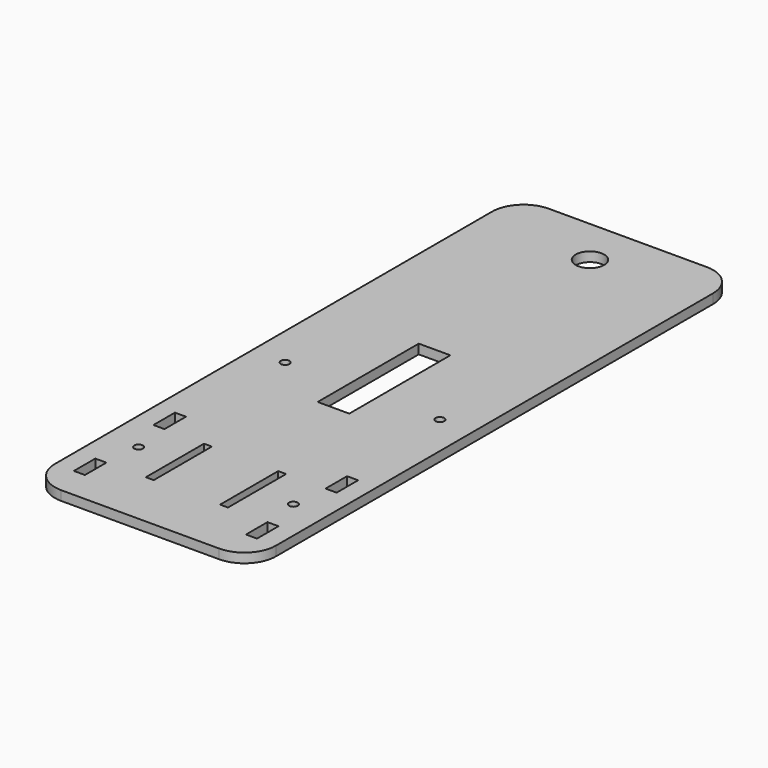
from build123d import *

# Parameters (mm, degrees)
F0_R     = 1.375
F0_R_2   = 4.5
F0_W     = 40
F0_H     = 10
F0_W_2   = 10
F0_H_2   = 35
F0_W_3   = 15
F0_H_3   = 2
F0_W_4   = 2
F0_W_5   = 5.5
F0_H_4   = 11.5
F0_R_3   = 1
F1_DEPTH = 3


# Not quite as in the source:
# - a feature names something its author has since deleted; it is built from what else it names


with BuildPart() as f1:
    # F0 (on Top) → F1 (new body)
    with BuildSketch(Plane.XY):
        with BuildLine():
            Line((25, 96.5), (-25, 96.5))
            ThreePointArc((-25, 96.5), (-32.0710678119, 93.5710678119), (-35, 86.5))
            Line((-35, 86.5), (-35, -86.5))
            ThreePointArc((-35, -86.5), (-32.0710678119, -93.5710678119), (-25, -96.5))
            Line((-25, -96.5), (25, -96.5))
            ThreePointArc((25, -96.5), (32.0710678119, -93.5710678119), (35, -86.5))
            Line((35, -86.5), (35, 86.5))
            ThreePointArc((35, 86.5), (32.0710678119, 93.5710678119), (25, 96.5))
        make_face()
        Polygon((-29, -86.5), (-29, -78), (-29, -55), (-29, -46.5), (-25.5, -46.5), (-25.5, -55), (-18.5, -55), (-13, -55), (-10.5, -55), (-10.5, -66.5), (-10.5, -78), (-10.5, -86.5), (-25.5, -86.5), align=None, mode=Mode.SUBTRACT)
        with Locations((-24.5, -8.5)):
            Circle(F0_R, mode=Mode.SUBTRACT)
        Polygon((10.5, -78), (10.5, -66.5), (10.5, -55), (13, -55), (18.5, -55), (24.5, -55), (25.5, -55), (25.5, -46.5), (29, -46.5), (29, -55), (29, -78), (29, -86.5), (25.5, -86.5), (10.5, -86.5), align=None, mode=Mode.SUBTRACT)
        with BuildLine():
            ThreePointArc((25.875, -8.5), (25.4722718241, -9.4722718241), (24.5, -9.875))
            ThreePointArc((24.5, -9.875), (23.5277281759, -7.5277281759), (25.875, -8.5))
        make_face(mode=Mode.SUBTRACT)
        with BuildLine():
            ThreePointArc((26, -30), (25.5980762114, -31.5), (24.5, -32.5980762114))
            ThreePointArc((24.5, -32.5980762114), (23.1822131445, -32.9944612821), (21.8260869565, -32.7607839768))
            ThreePointArc((21.8260869565, -32.7607839768), (0, -52), (-21.8260869565, -32.7607839768))
            ThreePointArc((-21.8260869565, -32.7607839768), (-26, -30), (-21.8260869565, -27.2392160232))
            ThreePointArc((-21.8260869565, -27.2392160232), (-16.3398685927, -15.268785034), (-5, -8.5757147144))
            Line((-5, -8.5757147144), (-5, -5.5))
            Line((-5, -5.5), (-14, -5.5))
            Line((-14, -5.5), (-14, -8.5))
            ThreePointArc((-14, -8.5), (-17, -11.5), (-20, -8.5))
            Line((-20, -8.5), (-20, -5.5))
            Line((-20, -5.5), (-30, -5.5))
            Line((-30, -5.5), (-32, -5.5))
            Line((-32, -5.5), (-32, 6.5))
            Line((-32, 6.5), (-32, 41.5))
            Line((-32, 41.5), (-32, 53.5))
            Line((-32, 53.5), (-30, 53.5))
            Line((-30, 53.5), (-30, 56.5))
            ThreePointArc((-30, 56.5), (-27, 59.5), (-24, 56.5))
            Line((-24, 56.5), (-24, 53.5))
            Line((-24, 53.5), (-20, 53.5))
            Line((-20, 53.5), (20, 53.5))
            Line((20, 53.5), (32, 53.5))
            Line((32, 53.5), (32, 41.5))
            Line((32, 41.5), (32, 6.5))
            Line((32, 6.5), (32, -5.5))
            Line((32, -5.5), (20, -5.5))
            Line((20, -5.5), (5, -5.5))
            Line((5, -5.5), (5, -8.5757147144))
            ThreePointArc((5, -8.5757147144), (16.3398685927, -15.268785034), (21.8260869565, -27.2392160232))
            ThreePointArc((21.8260869565, -27.2392160232), (23.1822131445, -27.0055387179), (24.5, -27.4019237886))
            ThreePointArc((24.5, -27.4019237886), (25.5980762114, -28.5), (26, -30))
        make_face(mode=Mode.SUBTRACT)
        with Locations((0, 81.5)):
            Circle(F0_R_2, mode=Mode.SUBTRACT)
        Polygon((5, 20), (5, 6.5), (20, 6.5), (20, 41.5), (-20, 41.5), (-20, 6.5), (-5, 6.5), (-5, 20), align=None)
        with BuildLine():
            ThreePointArc((-20, -30), (0, -50), (20, -30))
            ThreePointArc((20, -30), (15.8113883008, -17.7525512861), (5, -10.635083269))
            Line((5, -10.635083269), (5, -20))
            Line((5, -20), (-5, -20))
            Line((-5, -20), (-5, -10.635083269))
            ThreePointArc((-5, -10.635083269), (-15.8113883008, -17.7525512861), (-20, -30))
        make_face()
        with Locations((0, 46.5)):
            Rectangle(F0_W, F0_H)
        with Locations((-25, 24)):
            Rectangle(F0_W_2, F0_H_2)
        with Locations((25, 24)):
            Rectangle(F0_W_2, F0_H_2)
        Polygon((-29, -55), (-29, -78), (-25.5, -78), (-18.5, -78), (-18.5, -66.5), (-18.5, -55), (-25.5, -55), align=None)
        with Locations((-24.5, -66.5)):
            Circle(F0_R, mode=Mode.SUBTRACT)
        with BuildLine():
            Line((23.125, -66.5), (18.5, -66.5))
            Line((18.5, -66.5), (18.5, -78))
            Line((18.5, -78), (25.5, -78))
            Line((25.5, -78), (29, -78))
            Line((29, -78), (29, -55))
            Line((29, -55), (25.5, -55))
            Line((25.5, -55), (24.5, -55))
            Line((24.5, -55), (24.5, -65.125))
            ThreePointArc((24.5, -65.125), (25.4722718241, -65.5277281759), (25.875, -66.5))
            ThreePointArc((25.875, -66.5), (24.5, -67.875), (23.125, -66.5))
        make_face()
        with Locations((-12.5, 1.5)):
            Rectangle(F0_W_3, F0_H)
        with Locations((12.5, 1.5)):
            Rectangle(F0_W_3, F0_H)
        Polygon((-18.5, -78), (-25.5, -78), (-25.5, -86.5), (-10.5, -86.5), (-10.5, -78), (-13, -78), align=None)
        Polygon((13, -78), (10.5, -78), (10.5, -86.5), (25.5, -86.5), (25.5, -78), (18.5, -78), align=None)
        with BuildLine():
            ThreePointArc((-21.8260869565, -32.7607839768), (0, -52), (21.8260869565, -32.7607839768))
            ThreePointArc((21.8260869565, -32.7607839768), (20.4978270313, -31.6550318531), (20, -30))
            ThreePointArc((20, -30), (0, -50), (-20, -30))
            ThreePointArc((-20, -30), (-20.4978270313, -31.6550318531), (-21.8260869565, -32.7607839768))
        make_face()
        with Locations((25, 46.5)):
            Rectangle(F0_W_2, F0_H)
        with Locations((-25, 46.5)):
            Rectangle(F0_W_2, F0_H)
        with Locations((-25, 1.5)):
            Rectangle(F0_W_2, F0_H)
        with Locations((25, 1.5)):
            Rectangle(F0_W_2, F0_H)
        with Locations((0, 52.5)):
            Rectangle(F0_W, F0_H_3)
        with Locations((31, 24)):
            Rectangle(F0_W_4, F0_H_2)
        with Locations((-31, 24)):
            Rectangle(F0_W_4, F0_H_2)
        with BuildLine():
            Line((18.5, -55), (18.5, -66.5))
            Line((18.5, -66.5), (23.125, -66.5))
            ThreePointArc((23.125, -66.5), (23.5277281759, -65.5277281759), (24.5, -65.125))
            Line((24.5, -65.125), (24.5, -55))
            Line((24.5, -55), (18.5, -55))
        make_face()
        with Locations((-15.75, -72.25)):
            Rectangle(F0_W_5, F0_H_4)
        with Locations((-15.75, -60.75)):
            Rectangle(F0_W_5, F0_H_4)
        with Locations((15.75, -72.25)):
            Rectangle(F0_W_5, F0_H_4)
        with Locations((15.75, -60.75)):
            Rectangle(F0_W_5, F0_H_4)
        with BuildLine():
            ThreePointArc((-5, -8.5757147144), (-16.3398685927, -15.268785034), (-21.8260869565, -27.2392160232))
            ThreePointArc((-21.8260869565, -27.2392160232), (-20.4978270313, -28.3449681469), (-20, -30))
            ThreePointArc((-20, -30), (-15.8113883008, -17.7525512861), (-5, -10.635083269))
            Line((-5, -10.635083269), (-5, -8.5757147144))
        make_face()
        with BuildLine():
            ThreePointArc((20, -30), (20.4978270313, -28.3449681469), (21.8260869565, -27.2392160232))
            ThreePointArc((21.8260869565, -27.2392160232), (16.3398685927, -15.268785034), (5, -8.5757147144))
            Line((5, -8.5757147144), (5, -10.635083269))
            ThreePointArc((5, -10.635083269), (15.8113883008, -17.7525512861), (20, -30))
        make_face()
        Polygon((30, 41.5), (32, 41.5), (32, 53.5), (20, 53.5), (20, 51.5), (30, 51.5), align=None)
        Polygon((20, -3.5), (20, -5.5), (32, -5.5), (32, 6.5), (30, 6.5), (30, -3.5), align=None)
        Polygon((-14, -5.5), (-5, -5.5), (-5, -3.5), (-20, -3.5), (-20, -5.5), (-17, -5.5), align=None)
        with Locations((12.5, -4.5)):
            Rectangle(F0_W_3, F0_H_3)
        with BuildLine():
            ThreePointArc((-30, 56.5), (-29.1213203519, 54.3786796648), (-27.0000000236, 53.5))
            ThreePointArc((-27.0000000236, 53.5), (-24.8786796648, 54.3786796481), (-24, 56.5))
            ThreePointArc((-24, 56.5), (-27, 59.5), (-30, 56.5))
        make_face()
        with Locations((-27, 56.5)):
            Circle(F0_R_3, mode=Mode.SUBTRACT)
        with BuildLine():
            ThreePointArc((-14, -8.5), (-14.8786796564, -6.3786796564), (-17, -5.5))
            ThreePointArc((-17, -5.5), (-19.1213203436, -6.3786796564), (-20, -8.5))
            ThreePointArc((-20, -8.5), (-17, -11.5), (-14, -8.5))
        make_face()
        with Locations((-17, -8.5)):
            Circle(F0_R_3, mode=Mode.SUBTRACT)
        Polygon((-32, 41.5), (-30, 41.5), (-30, 51.5), (-30, 53.5), (-32, 53.5), align=None)
        Polygon((-30, -5.5), (-30, -3.5), (-30, 6.5), (-32, 6.5), (-32, -5.5), align=None)
        with BuildLine():
            ThreePointArc((-21.8260869565, -27.2392160232), (-26, -30), (-21.8260869565, -32.7607839768))
            ThreePointArc((-21.8260869565, -32.7607839768), (-21.9564786913, -31.3831281496), (-22, -30))
            ThreePointArc((-22, -30), (-21.9564786913, -28.6168718504), (-21.8260869565, -27.2392160232))
        make_face()
        with Locations((-23, -30)):
            Circle(F0_R_3, mode=Mode.SUBTRACT)
        Polygon((-30, 51.5), (-20, 51.5), (-20, 53.5), (-24, 53.5), (-27.0000000236, 53.5), (-30, 53.5), align=None)
        with Locations((-25, -4.5)):
            Rectangle(F0_W_2, F0_H_3)
        with BuildLine():
            ThreePointArc((21.8260869565, -32.7607839768), (23.1822131445, -32.9944612821), (24.5, -32.5980762114))
            Line((24.5, -32.5980762114), (24.5, -27.4019237886))
            ThreePointArc((24.5, -27.4019237886), (23.1822131445, -27.0055387179), (21.8260869565, -27.2392160232))
            ThreePointArc((21.8260869565, -27.2392160232), (21.9564786913, -28.6168718504), (22, -30))
            ThreePointArc((22, -30), (21.9564786913, -31.3831281496), (21.8260869565, -32.7607839768))
        make_face()
        with BuildLine():
            ThreePointArc((24, -30), (23, -31), (22, -30))
            ThreePointArc((22, -30), (23, -29), (24, -30))
        make_face(mode=Mode.SUBTRACT)
        with BuildLine():
            ThreePointArc((-22, -30), (-21.9564786913, -31.3831281496), (-21.8260869565, -32.7607839768))
            ThreePointArc((-21.8260869565, -32.7607839768), (-20.4978270313, -31.6550318531), (-20, -30))
            ThreePointArc((-20, -30), (-20.4978270313, -28.3449681469), (-21.8260869565, -27.2392160232))
            ThreePointArc((-21.8260869565, -27.2392160232), (-21.9564786913, -28.6168718504), (-22, -30))
        make_face()
        with BuildLine():
            ThreePointArc((20, -30), (20.4978270313, -31.6550318531), (21.8260869565, -32.7607839768))
            ThreePointArc((21.8260869565, -32.7607839768), (21.9564786913, -31.3831281496), (22, -30))
            ThreePointArc((22, -30), (21.9564786913, -28.6168718504), (21.8260869565, -27.2392160232))
            ThreePointArc((21.8260869565, -27.2392160232), (20.4978270313, -28.3449681469), (20, -30))
        make_face()
        with BuildLine():
            Line((24.5, -27.4019237886), (24.5, -32.5980762114))
            ThreePointArc((24.5, -32.5980762114), (25.5980762114, -31.5), (26, -30))
            ThreePointArc((26, -30), (25.5980762114, -28.5), (24.5, -27.4019237886))
        make_face()
        with Locations((-23, -30)):
            Circle(F0_R_3)
        with BuildLine():
            ThreePointArc((24, -30), (23, -29), (22, -30))
            ThreePointArc((22, -30), (23, -31), (24, -30))
        make_face()
        with Locations((-27, 56.5)):
            Circle(F0_R_3)
        with Locations((-17, -8.5)):
            Circle(F0_R_3)
        with BuildLine():
            Line((-27.0000000236, 53.5), (-24, 53.5))
            Line((-24, 53.5), (-24, 56.5))
            ThreePointArc((-24, 56.5), (-24.8786796648, 54.3786796481), (-27.0000000236, 53.5))
        make_face()
        with BuildLine():
            Line((-30, 56.5), (-30, 53.5))
            Line((-30, 53.5), (-27.0000000236, 53.5))
            ThreePointArc((-27.0000000236, 53.5), (-29.1213203519, 54.3786796648), (-30, 56.5))
        make_face()
        with BuildLine():
            ThreePointArc((-20, -8.5), (-19.1213203436, -6.3786796564), (-17, -5.5))
            Line((-17, -5.5), (-20, -5.5))
            Line((-20, -5.5), (-20, -8.5))
        make_face()
        with BuildLine():
            Line((-14, -8.5), (-14, -5.5))
            Line((-14, -5.5), (-17, -5.5))
            ThreePointArc((-17, -5.5), (-14.8786796564, -6.3786796564), (-14, -8.5))
        make_face()
    extrude(amount=F1_DEPTH)


solid = f1.part
